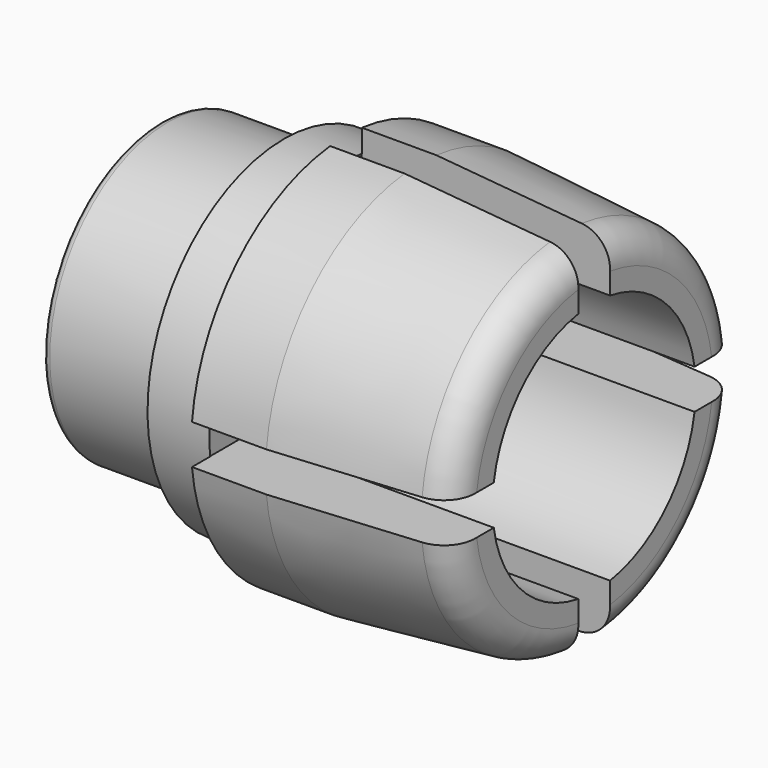
from build123d import *

# Parameters (mm, degrees)
F2_W          = 2.032
F2_H          = 3.556
F2_W_2        = 3.556
F2_H_2        = 2.032
F3_DEPTH      = 25.4
F3_DEPTH_BACK = 4.3434


# Not quite as in the source:
# - a feature names something its author has since deleted; it is built from what else it names


with BuildPart() as f1:
    # F0 (on Front) → F1 (revolve)
    with BuildSketch(Plane.XZ):
        with BuildLine():
            ThreePointArc((8.3732076521, 7.5855466623), (7.9877835669, 8.7130510839), (6.9264967271, 9.2547965866))
            Line((6.9264967271, 9.2547965866), (-0.5167923479, 9.906))
            Line((-0.5167923479, 9.906), (-4.3267923479, 9.906))
            Line((-4.3267923479, 9.906), (-4.3267923479, 8.73125))
            Line((-4.3267923479, 8.73125), (-7.5017923479, 8.73125))
            Line((-7.5017923479, 8.73125), (-7.5017923479, 7.5438))
            Line((-7.5017923479, 7.5438), (-13.4549173479, 7.5438))
            ThreePointArc((-13.4549173479, 7.5438), (-13.7355503517, 7.4275580038), (-13.8517923479, 7.146925))
            Line((-13.8517923479, 7.146925), (-13.8517923479, 6.5024))
            Line((-13.8517923479, 6.5024), (8.3732076521, 6.5024))
            Line((8.3732076521, 6.5024), (8.3732076521, 7.5855466623))
        make_face()
    revolve(axis=Axis((-0.2325048039, 0, 0), (1, 0, 0)))

    # F2 (on Right) → F3 (cut, two sides)
    with BuildSketch(Plane.YZ) as f3_sk:
        with Locations((0, -8.1534)):
            Rectangle(F2_W, F2_H)
        with Locations((0, 8.1534)):
            Rectangle(F2_W, F2_H)
        with Locations((-8.1534, 0)):
            Rectangle(F2_W_2, F2_H_2)
        with Locations((8.1534, 0)):
            Rectangle(F2_W_2, F2_H_2)
    extrude(amount=F3_DEPTH, mode=Mode.SUBTRACT)
    extrude(f3_sk.sketch, amount=-F3_DEPTH_BACK, mode=Mode.SUBTRACT)


solid = f1.part
